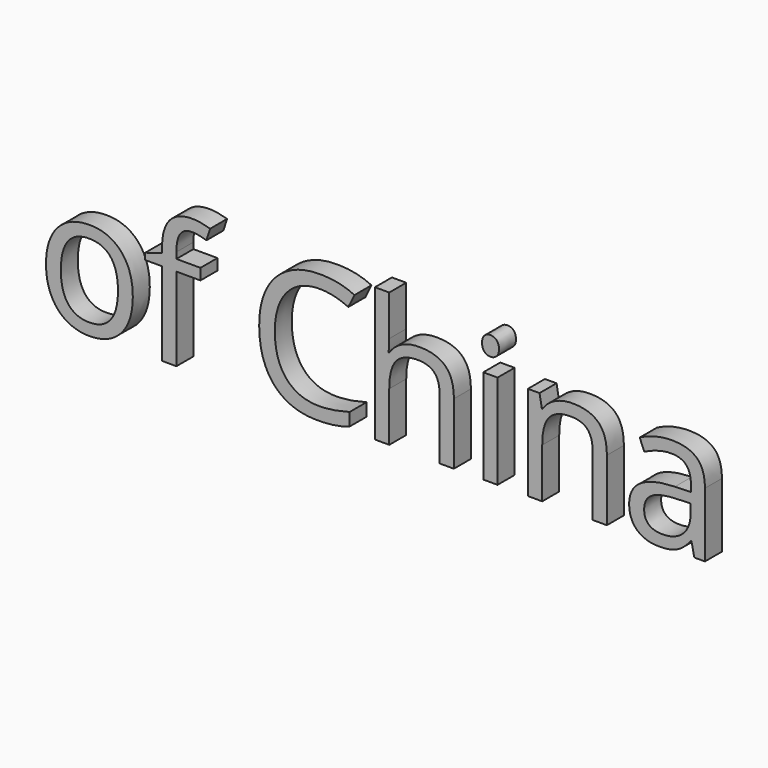
from build123d import *

# Parameters (mm, degrees)
F0_TEXT_SIZE = 211.1179340217
F1_DEPTH     = 25.4


# Not quite as in the source:
# - Text() gives the source's letters only with a copy of the font that has no kerning and outlines rounded to 1/6400 em; it was checked with that copy


with BuildPart() as f1:
    # F0 (on Front) → F1 (new body)
    with BuildSketch(Plane.XZ):
        with Locations((-75.1608833671, -75.3347203135)):
            Text('of China', F0_TEXT_SIZE, font='Open Sans', text_align=(TextAlign.LEFT, TextAlign.BOTTOM))
    extrude(amount=F1_DEPTH)


solid = f1.part
